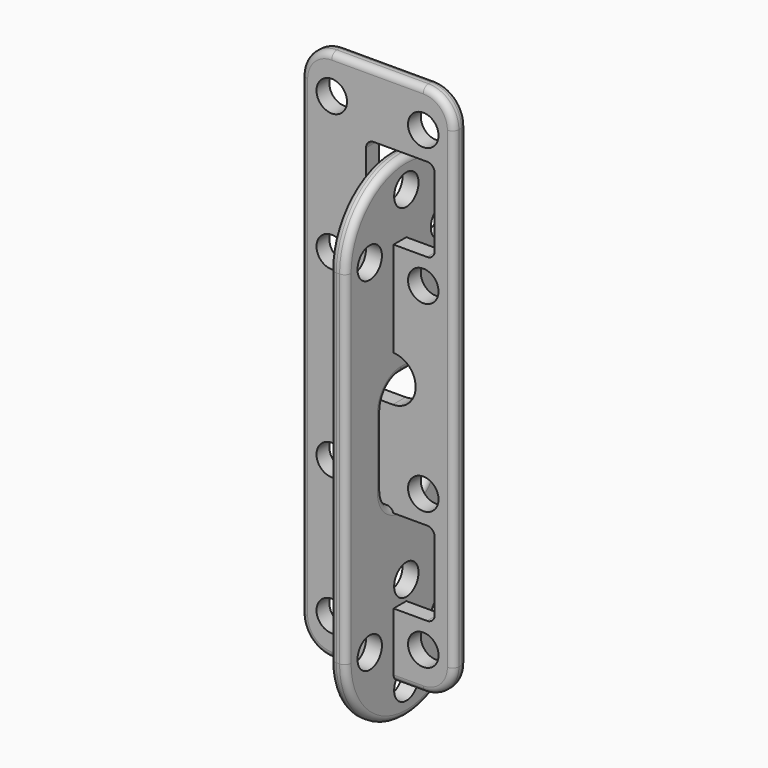
from build123d import *

# Parameters (mm, degrees)
F4_R      = 2
F5_DEPTH  = 2.1
F7_DEPTH  = 2.1
F8_R      = 0.84
F9_R      = 2
F10_DEPTH = 2.1
F11_R     = 0.84


# Not quite as in the source:
# - a feature names something its author has since deleted; it is built from what else it names


with BuildPart() as f5:
    # F4 (on Front) → F5 (new body)
    with BuildSketch(Plane.XZ):
        with BuildLine():
            ThreePointArc((10, 61), (8.8284271247, 63.8284271247), (6, 65))
            Line((6, 65), (-6, 65))
            ThreePointArc((-6, 65), (-8.8284271247, 63.8284271247), (-10, 61))
            Line((-10, 61), (-10, -1))
            ThreePointArc((-10, -1), (-8.8284271247, -3.8284271247), (-6, -5))
            Line((-6, -5), (6, -5))
            ThreePointArc((6, -5), (8.8284271247, -3.8284271247), (10, -1))
            Line((10, -1), (10, 61))
        make_face()
        with Locations((-6, 0)):
            Circle(F4_R, mode=Mode.SUBTRACT)
        with Locations((-6, 18)):
            Circle(F4_R, mode=Mode.SUBTRACT)
        with Locations((6, 0)):
            Circle(F4_R, mode=Mode.SUBTRACT)
        with Locations((6, 18)):
            Circle(F4_R, mode=Mode.SUBTRACT)
        with Locations((-6, 42)):
            Circle(F4_R, mode=Mode.SUBTRACT)
        with Locations((-6, 60)):
            Circle(F4_R, mode=Mode.SUBTRACT)
        with BuildLine():
            ThreePointArc((5, 30), (4.1213203436, 27.8786796564), (2, 27))
            Line((2, 27), (-2, 27))
            ThreePointArc((-2, 27), (-4.1213203436, 27.8786796564), (-5, 30))
            ThreePointArc((-5, 30), (-4.1213203436, 32.1213203436), (-2, 33))
            Line((-2, 33), (2, 33))
            ThreePointArc((2, 33), (4.1213203436, 32.1213203436), (5, 30))
        make_face(mode=Mode.SUBTRACT)
        with Locations((6, 42)):
            Circle(F4_R, mode=Mode.SUBTRACT)
        with Locations((6, 60)):
            Circle(F4_R, mode=Mode.SUBTRACT)
    extrude(amount=F5_DEPTH)

    # F6 (on Front) → F7 (cut, through all)
    with BuildSketch(Plane.XZ):
        with BuildLine():
            Line((6.5, 14.5), (-0.5, 14.5))
            ThreePointArc((-0.5, 14.5), (-1.2071067812, 14.2071067812), (-1.5, 13.5))
            Line((-1.5, 13.5), (-1.5, 4.5))
            ThreePointArc((-1.5, 4.5), (-1.2071067812, 3.7928932188), (-0.5, 3.5))
            Line((-0.5, 3.5), (6.5, 3.5))
            ThreePointArc((6.5, 3.5), (7.2071067812, 3.7928932188), (7.5, 4.5))
            Line((7.5, 4.5), (7.5, 13.5))
            ThreePointArc((7.5, 13.5), (7.2071067812, 14.2071067812), (6.5, 14.5))
        make_face()
        with BuildLine():
            ThreePointArc((-1.5, 46.5), (-1.2071067812, 45.7928932188), (-0.5, 45.5))
            Line((-0.5, 45.5), (6.5, 45.5))
            ThreePointArc((6.5, 45.5), (7.2071067812, 45.7928932188), (7.5, 46.5))
            Line((7.5, 46.5), (7.5, 55.5))
            ThreePointArc((7.5, 55.5), (7.2071067812, 56.2071067812), (6.5, 56.5))
            Line((6.5, 56.5), (-0.5, 56.5))
            ThreePointArc((-0.5, 56.5), (-1.2071067812, 56.2071067812), (-1.5, 55.5))
            Line((-1.5, 55.5), (-1.5, 46.5))
        make_face()
    extrude(amount=F7_DEPTH, mode=Mode.SUBTRACT)

    # F8
    f8_edges = [f5.edges().sort_by_distance(p)[0] for p in [
        (10, -1.05, -1),
        (10, -1.05, 61),
        (10, 0, 30),
        (10, -2.1, 30),
    ]]
    fillet(f8_edges, radius=F8_R)


with BuildPart() as f10:
    # F9 (on Right) → F10 (new body)
    with BuildSketch(Plane.YZ):
        with BuildLine():
            ThreePointArc((-9.9, 0), (0, -9.9), (9.9, 0))
            ThreePointArc((9.9, 0), (0, 9.9), (-9.9, 0))
        make_face()
        with Locations((-6, 0)):
            Circle(F9_R, mode=Mode.SUBTRACT)
        with Locations((0, -6)):
            Circle(F9_R, mode=Mode.SUBTRACT)
        Circle(F9_R, mode=Mode.SUBTRACT)
        with Locations((0, 6)):
            Circle(F9_R, mode=Mode.SUBTRACT)
        with Locations((6, 0)):
            Circle(F9_R, mode=Mode.SUBTRACT)
        with BuildLine():
            ThreePointArc((-9.9, 0), (0, 9.9), (9.9, 0))
            Line((9.9, 0), (9.9, 45))
            ThreePointArc((9.9, 45), (0, 35.1), (-9.9, 45))
            Line((-9.9, 45), (-9.9, 0))
        make_face()
        with BuildLine():
            ThreePointArc((3.9, 17.9), (3.0213203436, 15.7786796564), (0.9, 14.9))
            Line((0.9, 14.9), (-0.9, 14.9))
            ThreePointArc((-0.9, 14.9), (-3.0213203436, 15.7786796564), (-3.9, 17.9))
            Line((-3.9, 17.9), (-3.9, 27.1))
            ThreePointArc((-3.9, 27.1), (-3.0213203436, 29.2213203436), (-0.9, 30.1))
            Line((-0.9, 30.1), (0.9, 30.1))
            ThreePointArc((0.9, 30.1), (3.0213203436, 29.2213203436), (3.9, 27.1))
            Line((3.9, 27.1), (3.9, 17.9))
        make_face(mode=Mode.SUBTRACT)
        with BuildLine():
            ThreePointArc((-9.9, 45), (0, 35.1), (9.9, 45))
            ThreePointArc((9.9, 45), (0, 54.9), (-9.9, 45))
        make_face()
        with Locations((-6, 45)):
            Circle(F9_R, mode=Mode.SUBTRACT)
        with Locations((0, 39)):
            Circle(F9_R, mode=Mode.SUBTRACT)
        with Locations((0, 51)):
            Circle(F9_R, mode=Mode.SUBTRACT)
        with Locations((6, 45)):
            Circle(F9_R, mode=Mode.SUBTRACT)
    extrude(amount=F10_DEPTH)

    # F11
    f11_edges = [f10.edges().sort_by_distance(p)[0] for p in [
        (1.05, 9.9, 0),
        (1.05, 9.9, 45),
        (0, 9.9, 22.5),
        (2.1, 9.9, 22.5),
        (1.05, -3.9, 17.9),
        (1.05, -3.9, 27.1),
        (0, -3.9, 22.5),
        (2.1, -3.9, 22.5),
    ]]
    fillet(f11_edges, radius=F11_R)


solid = Compound([f5.part, f10.part])
